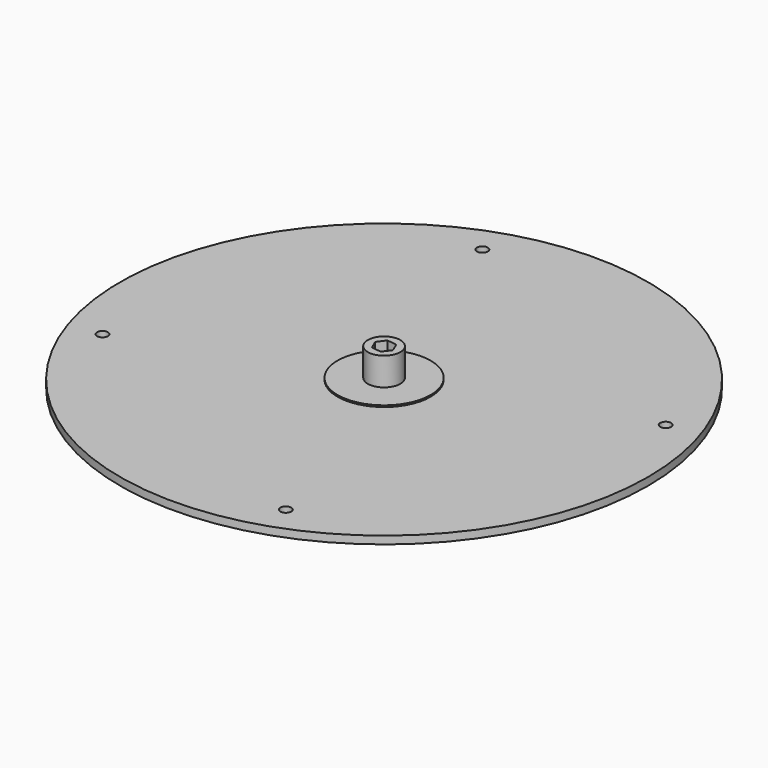
from build123d import *

# Parameters (mm, degrees)
F0_R            = 85
F0_R_2          = 1.75
F0_R_3          = 15
F0_R_4          = 5.25
F1_DEPTH        = 2.5
F2_DEPTH        = 2.5
F2_COPIES_COUNT = 4
F3_DEPTH        = 12
F4_DEPTH        = 9
F5_DEPTH        = 3


# Not quite as in the source:
# - a pattern or mirror of a feature is missing from the dataset's text; its kind, count and spacing are read off the source's solid


with BuildPart() as f1:
    # F0 (on Top) → F1 (new body)
    with BuildSketch(Plane.XY):
        Circle(F0_R)
        with Locations((-70.7297637461, -24.9459519848)):
            Circle(F0_R_2, mode=Mode.SUBTRACT)
        Circle(F0_R_3, mode=Mode.SUBTRACT)
        Circle(F0_R_3)
        Circle(F0_R_4, mode=Mode.SUBTRACT)
        Circle(F0_R_4)
        Polygon((-1.2691337593, 2.9107787333), (1.8862414482, 2.554491443), (3.1553752075, -0.3562872903), (1.2691337593, -2.9107787333), (-1.8862414482, -2.554491443), (-3.1553752075, 0.3562872903), align=None, mode=Mode.SUBTRACT)
        Polygon((3.1553752075, -0.3562872903), (1.8862414482, 2.554491443), (-1.2691337593, 2.9107787333), (-3.1553752075, 0.3562872903), (-1.8862414482, -2.554491443), (1.2691337593, -2.9107787333), align=None)
        Circle(F0_R_2, mode=Mode.SUBTRACT)
        with Locations((-70.7297637461, -24.9459519848)):
            Circle(F0_R_2)
    extrude(amount=F1_DEPTH)

    # F0 (on Top) → F2 (cut, through all)
    with BuildSketch(Plane.XY):
        with Locations((-70.7297637461, -24.9459519848)):
            Circle(F0_R_2)
    f2 = extrude(amount=F2_DEPTH, mode=Mode.SUBTRACT)

    # F2_copies: F2 ×4 about axis
    f2_copies_axis = Axis((0, 0, 0), (0, 0, 1))
    for i in range(1, F2_COPIES_COUNT):
        add(f2.rotate(f2_copies_axis, i * 360 / F2_COPIES_COUNT), mode=Mode.SUBTRACT)

    # F0 (on Top) → F3 (join)
    with BuildSketch(Plane.XY):
        Circle(F0_R_4)
        Polygon((-1.2691337593, 2.9107787333), (1.8862414482, 2.554491443), (3.1553752075, -0.3562872903), (1.2691337593, -2.9107787333), (-1.8862414482, -2.554491443), (-3.1553752075, 0.3562872903), align=None, mode=Mode.SUBTRACT)
    extrude(amount=F3_DEPTH)

    # F0 (on Top) → F4 (join)
    with BuildSketch(Plane.XY):
        Polygon((3.1553752075, -0.3562872903), (1.8862414482, 2.554491443), (-1.2691337593, 2.9107787333), (-3.1553752075, 0.3562872903), (-1.8862414482, -2.554491443), (1.2691337593, -2.9107787333), align=None)
        Circle(F0_R_2, mode=Mode.SUBTRACT)
    extrude(amount=F4_DEPTH)

    # F0 (on Top) → F5 (join)
    with BuildSketch(Plane.XY):
        Circle(F0_R_3)
        Circle(F0_R_4, mode=Mode.SUBTRACT)
    extrude(amount=F5_DEPTH)


solid = f1.part
